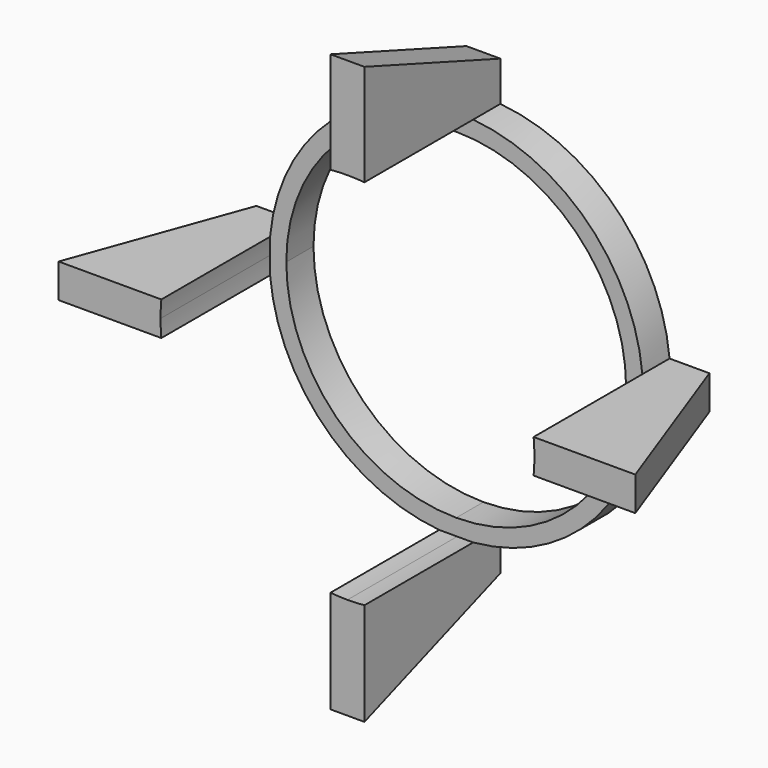
from build123d import *

# Parameters (mm, degrees)
F1_DEPTH    = 5.08
F2_DEPTH    = 25.4
F3_SIZE2    = 9.244834
F3_SIZE     = 25.39999
F4_T1_DEPTH = 139.04164749
F5_T1_DEPTH = 139.048329282
F6_SIZE2    = 9.244834
F6_SIZE     = 25.39999


# Not quite as in the source:
# - a fillet or chamfer that OpenCascade refuses, or shapes differently, is made with other operations: its cross-section is extruded or revolved along the edge and cut away or added
# - a fillet or chamfer is up to 0.001 mm smaller than in the source, because OpenCascade refuses the exact size


with BuildPart() as f1:
    # F0 (on Front) → F1 (new body)
    with BuildSketch(Plane.XZ):
        with BuildLine():
            Line((0, -27.8243059213), (0, -25.4))
            ThreePointArc((0, -25.4), (-17.9605122421, -17.9605122421), (-25.4, 0))
            Line((-25.4, 0), (-27.8243059213, 0))
            Line((-27.8243059213, 0), (-27.8243059213, -2.54))
            ThreePointArc((-27.8243059213, -2.54), (-19.7565634664, -19.7565634664), (-2.54, -27.8243059213))
            Line((-2.54, -27.8243059213), (0, -27.8243059213))
        make_face()
        with BuildLine():
            Line((27.8243059213, 0), (25.4, 0))
            ThreePointArc((25.4, 0), (17.9605122421, -17.9605122421), (0, -25.4))
            Line((0, -25.4), (0, -27.8243059213))
            Line((0, -27.8243059213), (2.54, -27.8243059213))
            ThreePointArc((2.54, -27.8243059213), (19.7565634664, -19.7565634664), (27.8243059213, -2.54))
            Line((27.8243059213, -2.54), (27.8243059213, 0))
        make_face()
        with BuildLine():
            ThreePointArc((0, 25.4), (17.9605122421, 17.9605122421), (25.4, 0))
            Line((25.4, 0), (27.8243059213, 0))
            Line((27.8243059213, 0), (27.8243059213, 2.54))
            ThreePointArc((27.8243059213, 2.54), (19.7541911569, 19.758935491), (2.533318208, 27.8249150737))
            Line((2.533318208, 27.8249150737), (0, 27.8249150737))
            Line((0, 27.8249150737), (0, 27.8243059213))
            Line((0, 27.8243059213), (0, 25.4))
        make_face()
        with BuildLine():
            ThreePointArc((-25.4, 0), (-17.9605122421, 17.9605122421), (0, 25.4))
            Line((0, 25.4), (0, 27.8243059213))
            Line((0, 27.8243059213), (-2.54, 27.8243059213))
            ThreePointArc((-2.54, 27.8243059213), (-19.7565634664, 19.7565634664), (-27.8243059213, 2.54))
            Line((-27.8243059213, 2.54), (-27.8243059213, 0))
            Line((-27.8243059213, 0), (-25.4, 0))
        make_face()
    extrude(amount=F1_DEPTH)


with BuildPart() as f2:
    # F0 (on Front) → F2 (new body)
    with BuildSketch(Plane.XZ):
        with BuildLine():
            ThreePointArc((-27.8243059213, -2.54), (-27.911061494, -1.2713167504), (-27.94, 0))
            Line((-27.94, 0), (-43.18, 0))
            Line((-43.18, 0), (-43.18, -2.54))
            Line((-43.18, -2.54), (-27.8243059213, -2.54))
        make_face()
        with BuildLine():
            Line((-43.18, 0), (-27.94, 0))
            ThreePointArc((-27.94, 0), (-27.911061494, 1.2713167504), (-27.8243059213, 2.54))
            Line((-27.8243059213, 2.54), (-43.18, 2.54))
            Line((-43.18, 2.54), (-43.18, 0))
        make_face()
    extrude(amount=F2_DEPTH)

    # F3 (size 25.4 and 9.2448439504 in the source; OpenCascade refuses exactly that, so slightly less here)
    f3_edges = [f2.edges().sort_by_distance(p)[0] for p in [
        (-43.18, 0, 0),
    ]]
    chamfer(f3_edges, length=F3_SIZE, length2=F3_SIZE2)


with BuildPart() as f2b:
    # F0 (on Front) → F2, piece 2 (new body)
    with BuildSketch(Plane.XZ):
        with BuildLine():
            ThreePointArc((0, 27.94), (1.2679654651, 27.9112139395), (2.533318208, 27.8249150737))
            Line((2.533318208, 27.8249150737), (2.533318208, 43.18))
            Line((2.533318208, 43.18), (0, 43.18))
            Line((0, 43.18), (0, 27.94))
        make_face()
        with BuildLine():
            Line((-2.54, 43.18), (-2.54, 27.8243059213))
            ThreePointArc((-2.54, 27.8243059213), (-1.2713167504, 27.911061494), (0, 27.94))
            Line((0, 27.94), (0, 43.18))
            Line((0, 43.18), (-2.54, 43.18))
        make_face()
    extrude(amount=F2_DEPTH)

    # F4: chamfer of 9.398 x 25.820792788 on 1 edges, made by hand

    # F4_s2 → F4_t1 (cut)
    with BuildSketch(Plane.YZ.offset(-69.524164641)):
        Polygon((-25.820792788, 43.18), (0, 33.782), (0, 43.18), align=None)
    extrude(amount=F4_T1_DEPTH, mode=Mode.SUBTRACT)


with BuildPart() as f2c:
    # F0 (on Front) → F2, piece 3 (new body)
    with BuildSketch(Plane.XZ):
        with BuildLine():
            Line((43.18, 0), (27.94, 0))
            ThreePointArc((27.94, 0), (27.911061494, -1.2713167504), (27.8243059213, -2.54))
            Line((27.8243059213, -2.54), (43.18, -2.54))
            Line((43.18, -2.54), (43.18, 0))
        make_face()
        with BuildLine():
            ThreePointArc((27.8243059213, 2.54), (27.911061494, 1.2713167504), (27.94, 0))
            Line((27.94, 0), (43.18, 0))
            Line((43.18, 0), (43.18, 2.54))
            Line((43.18, 2.54), (27.8243059213, 2.54))
        make_face()
    extrude(amount=F2_DEPTH)

    # F5: chamfer of 9.398 x 25.820792788 on 1 edges, made by hand

    # F5_s2 → F5_t1 (cut)
    with BuildSketch(Plane.XY.offset(-69.524164641)):
        Polygon((43.18, -25.820792788), (33.782, 0), (43.18, 0), align=None)
    extrude(amount=F5_T1_DEPTH, mode=Mode.SUBTRACT)


with BuildPart() as f2d:
    # F0 (on Front) → F2, piece 4 (new body)
    with BuildSketch(Plane.XZ):
        with BuildLine():
            ThreePointArc((2.54, -27.8243059213), (1.2713167504, -27.911061494), (0, -27.94))
            Line((0, -27.94), (0, -43.18))
            Line((0, -43.18), (2.54, -43.18))
            Line((2.54, -43.18), (2.54, -27.8243059213))
        make_face()
        with BuildLine():
            Line((0, -43.18), (0, -27.94))
            ThreePointArc((0, -27.94), (-1.2713167504, -27.911061494), (-2.54, -27.8243059213))
            Line((-2.54, -27.8243059213), (-2.54, -43.18))
            Line((-2.54, -43.18), (0, -43.18))
        make_face()
    extrude(amount=F2_DEPTH)

    # F6 (size 25.4 and 9.2448439504 in the source; OpenCascade refuses exactly that, so slightly less here)
    f6_edges = [f2d.edges().sort_by_distance(p)[0] for p in [
        (0, 0, -43.18),
    ]]
    f6_side = f2d.faces().sort_by_distance((0, -12.7, -43.18))[0]
    chamfer(f6_edges, length=F6_SIZE, length2=F6_SIZE2, reference=f6_side)


solid = Compound([f1.part, f2.part, f2b.part, f2c.part, f2d.part])
